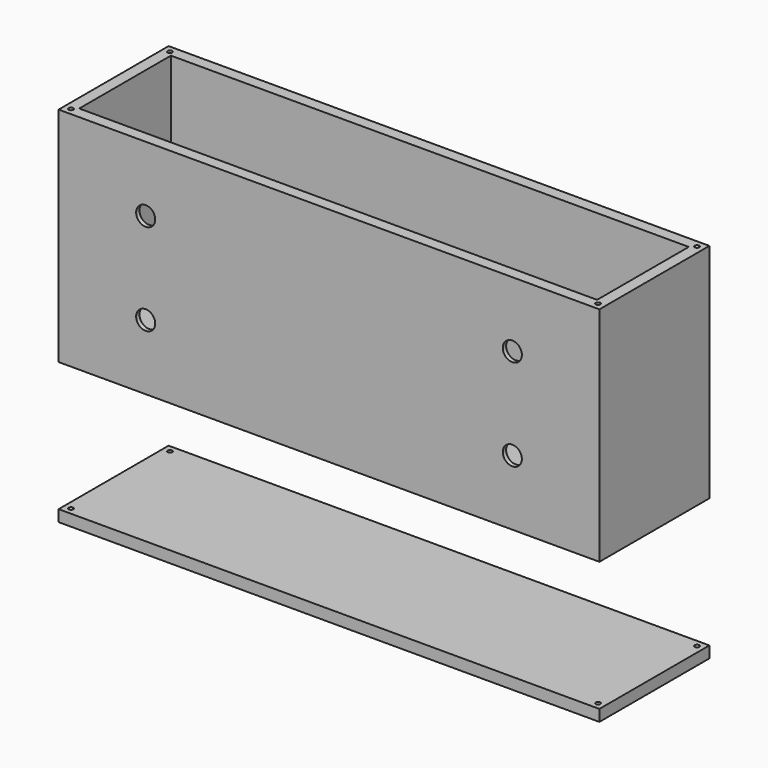
from build123d import *

# Parameters (mm, degrees)
F0_W      = 118
F0_H      = 48.5
F1_DEPTH  = 15
F2_T      = -2.5
F3_W      = 22
F3_H      = 5
F4_DEPTH  = 59.4
F5_R      = 2.0828
F6_DEPTH  = 25
F8_W      = 118
F8_H      = 30
F9_DEPTH  = 2.5
F10_R     = 0.5
F11_DEPTH = 55
F12_R     = 0.5
F13_DEPTH = 5
F14_R     = 5.159375
F15_DEPTH = 1.5875


# Not quite as in the source:
# - a length typed as a fraction of an inch, garbled in the dataset ("3 / 203.2 mm" for 3/8 in), is restored


with BuildPart() as f1:
    # F0 (on Front) → F1 (new body, symmetric)
    with BuildSketch(Plane.XZ):
        Rectangle(F0_W, F0_H)
    extrude(amount=F1_DEPTH, both=True)

    # F2
    f2_openings = [f1.faces().sort_by_distance(p)[0] for p in [
        (0, 0, 24.25),
    ]]
    offset(amount=F2_T, openings=f2_openings)

    # F3 (on Right) → F4 (cut)
    with BuildSketch(Plane.YZ):
        with Locations((0, -19.25)):
            Rectangle(F3_W, F3_H)
    extrude(amount=-F4_DEPTH, mode=Mode.SUBTRACT)

    # F5 (on Front) → F6 (cut)
    with BuildSketch(Plane.XZ):
        with Locations((40, -10)):
            Circle(F5_R)
        with Locations((-40, -10)):
            Circle(F5_R)
        with Locations((-40, 10)):
            Circle(F5_R)
        with Locations((40, 10)):
            Circle(F5_R)
    extrude(amount=F6_DEPTH, mode=Mode.SUBTRACT)

    # F12 (on face) → F13 (cut)
    with BuildSketch(Plane.XY.offset(24.25)):
        with Locations((-57.5, 13.5)):
            Circle(F12_R)
        with Locations((-57.5, -13.5)):
            Circle(F12_R)
        with Locations((57.5, -13.5)):
            Circle(F12_R)
        with Locations((57.5, 13.5)):
            Circle(F12_R)
    extrude(amount=-F13_DEPTH, mode=Mode.SUBTRACT)

    # F14 (on face) → F15 (cut)
    with BuildSketch(Plane(origin=(0, -12.5, 0), x_dir=(-1, 0, 0), z_dir=(0, 1, 0))):
        with Locations((40, -10)):
            Circle(F14_R)
        with Locations((40, 10)):
            Circle(F14_R)
        with Locations((-40, 10)):
            Circle(F14_R)
        with Locations((-40, -10)):
            Circle(F14_R)
    extrude(amount=-F15_DEPTH, mode=Mode.SUBTRACT)


with BuildPart() as f9:
    # F8 (on offset) → F9 (new body)
    with BuildSketch(Plane.XY.offset(-55)):
        Rectangle(F8_W, F8_H)
    extrude(amount=F9_DEPTH)

    # F10 (on offset) → F11 (cut)
    with BuildSketch(Plane.XY.offset(-55)):
        with Locations((-57.5, 13.5)):
            Circle(F10_R)
        with Locations((-57.5, -13.5)):
            Circle(F10_R)
        with Locations((57.5, -13.5)):
            Circle(F10_R)
        with Locations((57.5, 13.5)):
            Circle(F10_R)
    extrude(amount=F11_DEPTH, mode=Mode.SUBTRACT)


solid = Compound([f1.part, f9.part])
